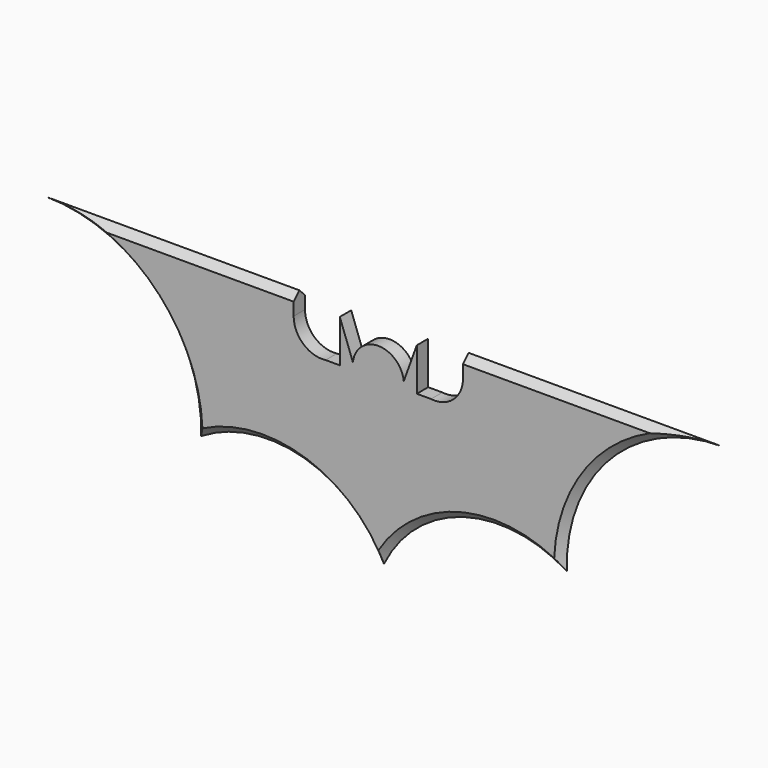
from build123d import *

# Parameters (mm, degrees)
F1_DEPTH = 1.27
F2_SIZE  = 1.26999


# Not quite as in the source:
# - a fillet or chamfer is up to 0.001 mm smaller than in the source, because OpenCascade refuses the exact size
# - a feature names something its author has since deleted; it is built from what else it names


with BuildPart() as f1:
    # F0 (on Front) → F1 (new body, symmetric)
    with BuildSketch(Plane.XZ):
        with BuildLine():
            Line((-15.113, 14.986), (-60.325, 14.986))
            ThreePointArc((-60.325, 14.986), (-40.4178225843, 6.541072822), (-32.6550259817, -13.6418778197))
            ThreePointArc((-32.6550259817, -13.6418778197), (-14.2166113122, -11.1006310534), (0, -23.114))
            ThreePointArc((0, -23.114), (14.2166113122, -11.1006310534), (32.6550259817, -13.6418778197))
            ThreePointArc((32.6550259817, -13.6418778197), (40.4178225843, 6.541072822), (60.325, 14.986))
            Line((60.325, 14.986), (15.113, 14.986))
            Line((15.113, 14.986), (15.113, 11.43))
            ThreePointArc((15.113, 11.43), (13.3972241951, 7.623637489), (9.4089072578, 6.3884815532))
            Line((9.4089072578, 6.3884815532), (6.8689072578, 6.3884815532))
            Line((6.8689072578, 6.3884815532), (6.8689072578, 14.0084815532))
            Line((6.8689072578, 14.0084815532), (4.5436901303, 7.62))
            ThreePointArc((4.5436901303, 7.62), (0, 11.684), (-4.5436901303, 7.62))
            Line((-4.5436901303, 7.62), (-6.8689072578, 14.0084815532))
            Line((-6.8689072578, 14.0084815532), (-6.8689072578, 6.3884815532))
            Line((-6.8689072578, 6.3884815532), (-9.4089072578, 6.3884815532))
            ThreePointArc((-9.4089072578, 6.3884815532), (-13.3972241951, 7.623637489), (-15.113, 11.43))
            Line((-15.113, 11.43), (-15.113, 14.986))
        make_face()
    extrude(amount=F1_DEPTH, both=True)

    # F2 (size 1.27 in the source; OpenCascade refuses exactly that, so slightly less here)
    f2_edges = [f1.edges().sort_by_distance(p)[0] for p in [
        (-40.417823, -1.27, 6.541073),
        (-37.719, -1.27, 14.986),
        (-14.216611, -1.27, -11.100631),
        (-14.216611, 1.27, -11.100631),
        (-40.417823, 1.27, 6.541073),
        (-37.719, 1.27, 14.986),
        (37.719, -1.27, 14.986),
        (40.417823, -1.27, 6.541073),
        (14.216611, -1.27, -11.100631),
        (37.719, 1.27, 14.986),
        (40.417823, 1.27, 6.541073),
        (14.216611, 1.27, -11.100631),
    ]]
    chamfer(f2_edges, length=F2_SIZE)


solid = f1.part
